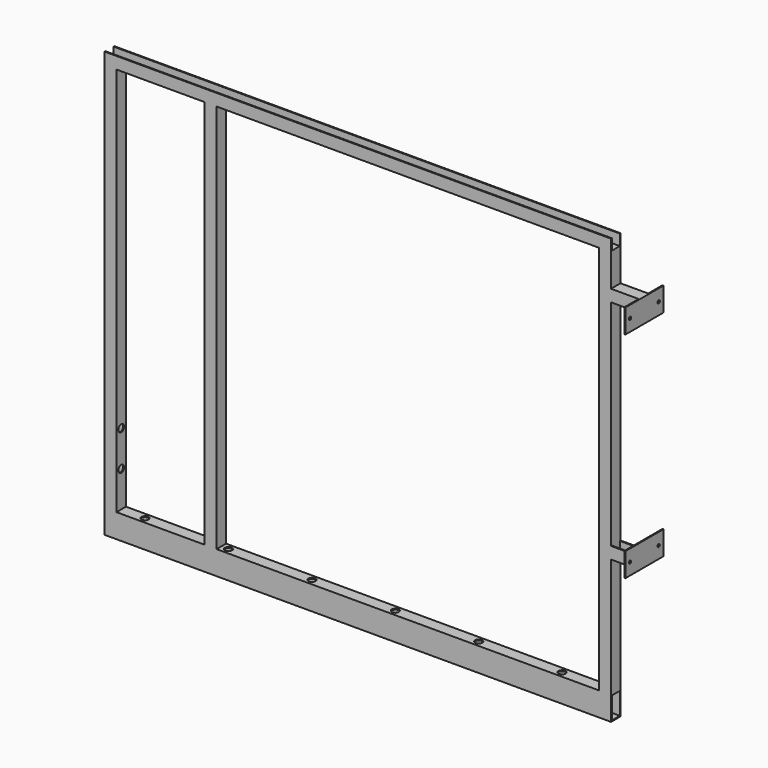
from build123d import *

# Parameters (mm, degrees)
F0_W      = 42
F0_H      = 42
F1_DEPTH  = 1635
F2_W      = 42
F2_H      = 92
F3_DEPTH  = 2125
F7_DEPTH  = 2125
F8_R      = 15
F9_DEPTH  = 50
F10_R     = 15
F11_DEPTH = 250
F13_DEPTH = 116
F14_W     = 200
F14_H     = 100
F14_R     = 6
F15_DEPTH = 4
F16_W     = 50
F16_H     = 50
F16_W_2   = 42
F16_H_2   = 42
F17_DEPTH = 1635
F18_R     = 7
F19_DEPTH = 125
F20_R     = 15
F20_R_2   = 7
F21_DEPTH = 5


# Not quite as in the source:
# - a feature names something its author has since deleted; it is built from what else it names


with BuildPart() as f1:
    # F0 (on Top) → F1 (new body)
    with BuildSketch(Plane.XY):
        Polygon((0, 4), (0, 0), (50, 0), (50, 50), (0, 50), (0, 46), align=None)
        with Locations((25, 25)):
            Rectangle(F0_W, F0_H, mode=Mode.SUBTRACT)
    extrude(amount=F1_DEPTH)


with BuildPart() as f3:
    # F2 (on face) → F3 (new body)
    with BuildSketch(Plane(origin=(0, 0, 0), x_dir=(0, -1, 0), z_dir=(-1, 0, 0))):
        Polygon((0, 0), (-50, 0), (-50, -4), (-50, -96), (-50, -100), (0, -100), align=None)
        with Locations((-25, -50)):
            Rectangle(F2_W, F2_H, mode=Mode.SUBTRACT)
    extrude(amount=-F3_DEPTH)

    # F5: F1 across plane
    add(f1.part.mirror(Plane.YZ.offset(1062.5)))


with BuildPart() as f1_1:
    add(f1.part)

    add(f3.part)  # F7 merges F3
    # F6 (on face) → F7 (join, through all)
    with BuildSketch(Plane(origin=(0, 0, 0), x_dir=(0, -1, 0), z_dir=(-1, 0, 0))):
        Polygon((-46, 1685), (-50, 1685), (-50, 1635), (0, 1635), (0, 1685), (-4, 1685), (-4, 1639), (-46, 1639), align=None)
    extrude(amount=-F7_DEPTH)

    # F8 (on face) → F9 (cut)
    with BuildSketch(Plane.XY.offset(1639)):
        with Locations((315, 25)):
            Circle(F8_R)
        with Locations((155, 25)):
            Circle(F8_R)
        with Locations((255, 25)):
            Circle(F8_R)
        with Locations((95, 25)):
            Circle(F8_R)
    extrude(amount=-F9_DEPTH, mode=Mode.SUBTRACT)

    # F10 (on face) → F11 (cut)
    with BuildSketch(Plane.YZ.offset(50)):
        with Locations((25, 300)):
            Circle(F10_R)
        with Locations((25, 150)):
            Circle(F10_R)
    extrude(amount=-F11_DEPTH, mode=Mode.SUBTRACT)

    # F12 (on face) → F13 (join)
    with BuildSketch(Plane.YZ.offset(2125)):
        Polygon((4, 550), (0, 550), (0, 500), (50, 500), (50, 550), (46, 550), (46, 504), (4, 504), align=None)
        Polygon((0, 1500), (0, 1450), (4, 1450), (4, 1496), (46, 1496), (46, 1450), (50, 1450), (50, 1500), align=None)
    extrude(amount=F13_DEPTH)

    # F14 (on face) → F15 (join)
    with BuildSketch(Plane.YZ.offset(2241)):
        with Locations((25, 1450)):
            Rectangle(F14_W, F14_H)
        with Locations((-50, 1450)):
            Circle(F14_R, mode=Mode.SUBTRACT)
        with Locations((100, 1450)):
            Circle(F14_R, mode=Mode.SUBTRACT)
        with Locations((25, 550)):
            Rectangle(F14_W, F14_H)
        with Locations((-50, 550)):
            Circle(F14_R, mode=Mode.SUBTRACT)
        with Locations((100, 550)):
            Circle(F14_R, mode=Mode.SUBTRACT)
    extrude(amount=F15_DEPTH)

    # F16 (on face) → F17 (join, through all)
    with BuildSketch(Plane.XY):
        with Locations((445, 25)):
            Rectangle(F16_W, F16_H)
        with Locations((445, 25)):
            Rectangle(F16_W_2, F16_H_2, mode=Mode.SUBTRACT)
    extrude(amount=F17_DEPTH)

    # F18 (on face) → F19 (cut)
    with BuildSketch(Plane(origin=(0, 0, -100), x_dir=(1, 0, 0), z_dir=(0, 0, -1))):
        with Locations((150, -25)):
            Circle(F18_R)
        with Locations((500, -25)):
            Circle(F18_R)
        with Locations((850, -25)):
            Circle(F18_R)
        with Locations((1200, -25)):
            Circle(F18_R)
        with Locations((1550, -25)):
            Circle(F18_R)
        with Locations((1900, -25)):
            Circle(F18_R)
    extrude(amount=-F19_DEPTH, mode=Mode.SUBTRACT)

    # F20 (on face) → F21 (cut)
    with BuildSketch(Plane.XY):
        with Locations((500, 25)):
            Circle(F20_R)
        with Locations((500, 25)):
            Circle(F20_R_2, mode=Mode.SUBTRACT)
        with Locations((850, 25)):
            Circle(F20_R)
        with Locations((850, 25)):
            Circle(F20_R_2, mode=Mode.SUBTRACT)
        with Locations((1200, 25)):
            Circle(F20_R)
        with Locations((1200, 25)):
            Circle(F20_R_2, mode=Mode.SUBTRACT)
        with Locations((1550, 25)):
            Circle(F20_R)
        with Locations((1550, 25)):
            Circle(F20_R_2, mode=Mode.SUBTRACT)
        with Locations((1900, 25)):
            Circle(F20_R)
        with Locations((1900, 25)):
            Circle(F20_R_2, mode=Mode.SUBTRACT)
        with Locations((150, 25)):
            Circle(F20_R)
    extrude(amount=-F21_DEPTH, mode=Mode.SUBTRACT)


solid = f1_1.part
